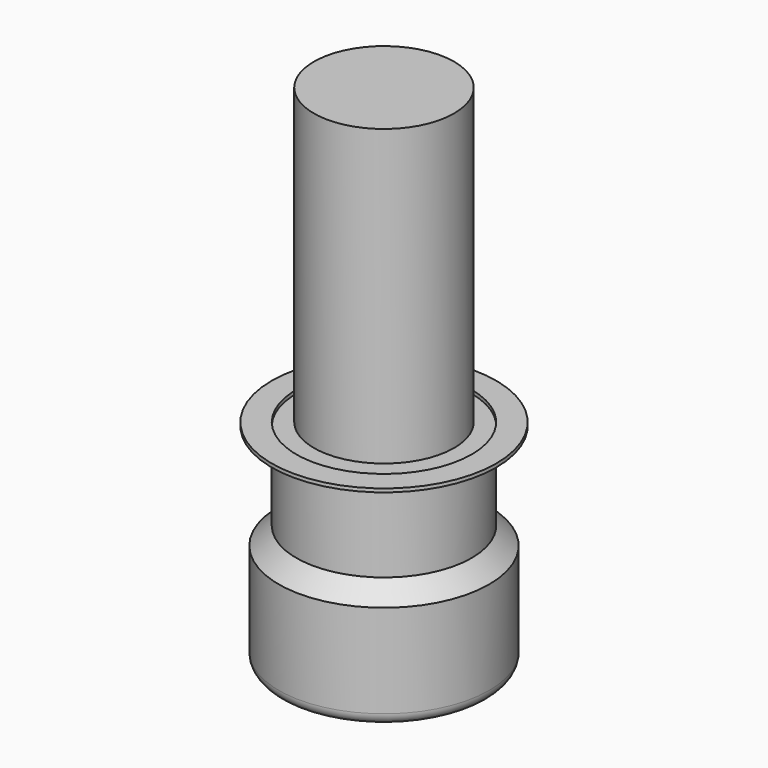
from build123d import *

# Parameters (mm, degrees)
F0_R        = 15
F1_DEPTH    = 20
F2_R        = 12.5
F3_DEPTH    = 10
F4_R        = 16
F4_R_2      = 12.5
F5_DEPTH    = 0.5
F6_R        = 10
F7_DEPTH    = 42
F8_R        = 1.6899494937
F9_S5_R     = 12.5
F9_T6_DEPTH = 23


# Not quite as in the source:
# - a fillet or chamfer that OpenCascade refuses, or shapes differently, is made with other operations: its cross-section is extruded or revolved along the edge and cut away or added


with BuildPart() as f1:
    # F0 (on Top) → F1 (new body)
    with BuildSketch(Plane.XY):
        Circle(F0_R)
    extrude(amount=F1_DEPTH)

    # F2 (on face) → F3 (join)
    with BuildSketch(Plane.XY.offset(20)):
        Circle(F2_R)
    extrude(amount=F3_DEPTH)

    # F8
    f8_edges = [f1.edges().sort_by_distance(p)[0] for p in [
        (-15, 0, 0),
    ]]
    fillet(f8_edges, radius=F8_R)

    # F9: chamfer of 5 on 1 edges, made by hand


with BuildPart() as f5:
    # F4 (on face) → F5 (new body)
    with BuildSketch(Plane.XY.offset(30)):
        Circle(F4_R)
        Circle(F4_R_2, mode=Mode.SUBTRACT)
    extrude(amount=F5_DEPTH)


with BuildPart() as f7:
    # F6 (on face) → F7 (new body)
    with BuildSketch(Plane.XY.offset(30.5)):
        Circle(F6_R)
    extrude(amount=F7_DEPTH)


with BuildPart() as f9_tool2:
    # F9_s3 → F9_t4 (revolve)
    with BuildSketch(Plane.XZ):
        Polygon((15, 15), (10, 20), (15, 20), align=None)
    revolve(axis=Axis((0, 0, 20), (0, 0, 1)))

    # F9_s5 → F9_t6 (cut, symmetric)
    with BuildSketch(Plane.XY.offset(17.5)):
        Circle(F9_S5_R)
    extrude(amount=F9_T6_DEPTH, both=True, mode=Mode.SUBTRACT)


with BuildPart() as f1_1:
    add(f1.part)

    # F9_t1: cut F9_tool2
    add(f9_tool2.part, mode=Mode.SUBTRACT)


solid = Compound([f5.part, f7.part, f1_1.part])
